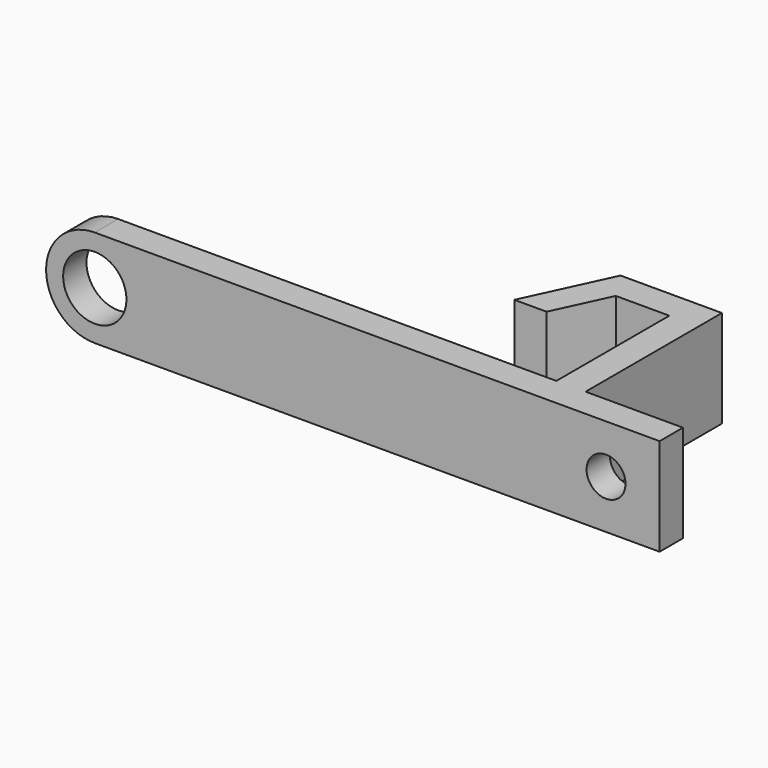
from build123d import *

# Parameters (mm, degrees)
F0_W     = 50
F0_H     = 3
F1_DEPTH = 10
F3_D     = 4
F5_R     = 4.99999
F6_D     = 6.5


# Not quite as in the source:
# - a fillet or chamfer is up to 0.001 mm smaller than in the source, because OpenCascade refuses the exact size


with BuildPart() as f1:
    # F0 (on Top) → F1 (new body)
    with BuildSketch(Plane.XY):
        Polygon((-2.2981421612, -11.8900760232), (10.7018578388, -11.8900760232), (10.7018578388, -8.8900760232), (0.7018578388, -8.8900760232), (0.7018578388, 8.6099239768), (-9.7093529436, 8.6099239768), (-13.7242264302, 0), (-10.4140926733, 0), (-7.7981421612, 5.6099239768), (-2.2981421612, 5.6099239768), (-2.2981421612, -8.8900760232), align=None)
        with Locations((-27.2981421612, -10.3900760232)):
            Rectangle(F0_W, F0_H)
    extrude(amount=F1_DEPTH)

    # F3 (through all)
    with Locations(Plane(origin=(0, -8.8900760232, 0), x_dir=(-1, 0, 0), z_dir=(0, 1, 0))):
        with Locations((-5.2018578388, 5)):
            Hole(F3_D / 2)

    # F5 (radius 5 in the source; OpenCascade refuses exactly that, so slightly less here)
    f5_edges = [f1.edges().sort_by_distance(p)[0] for p in [
        (-52.298142, -10.390076, 10),
        (-52.298142, -10.390076, 0),
    ]]
    fillet(f5_edges, radius=F5_R)

    # F6 (through all)
    with Locations(Plane.XZ.offset(11.8900760232)):
        with Locations((-47.2981421612, 5)):
            Hole(F6_D / 2)


solid = f1.part
